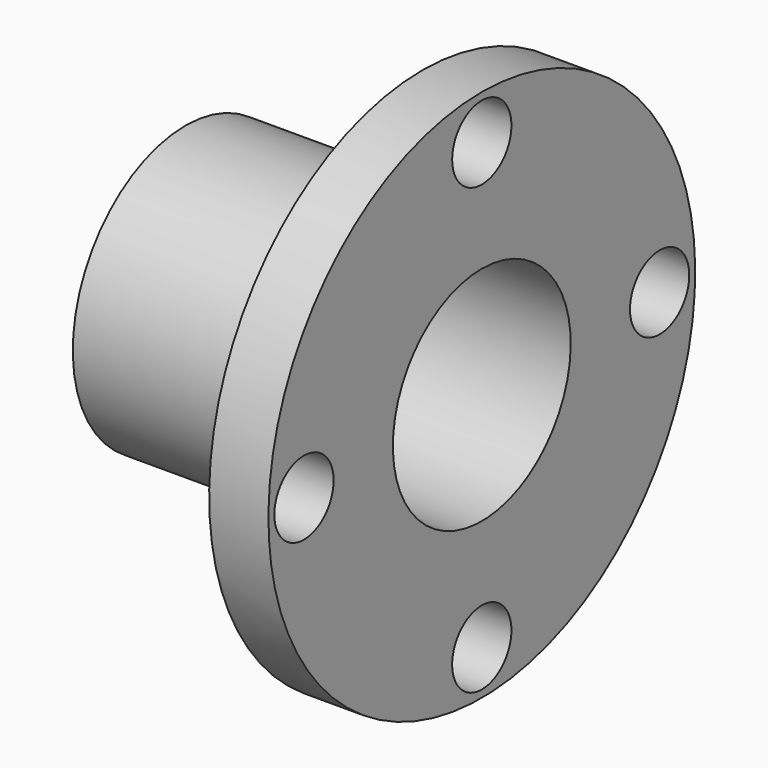
from build123d import *

# Parameters (mm, degrees)
F2_R            = 12.5
F3_DEPTH        = 20.001
F3_COPIES_COUNT = 4


# Not quite as in the source:
# - a pattern or mirror of a feature is missing from the dataset's text; its kind, count and spacing are read off the source's solid


with BuildPart() as f1:
    # F0 (on Front) → F1 (revolve)
    with BuildSketch(Plane.XZ):
        Polygon((-100, 37.5), (0, 37.5), (0, 90), (-20, 90), (-20, 47.5), (-100, 47.5), align=None)
    revolve(axis=Axis((-86.3388044803, 0, 0), (-1, 0, 0)))

    # F2 (on face) → F3 (cut, through all)
    with BuildSketch(Plane(origin=(-20, 0, 0), x_dir=(0, -1, 0), z_dir=(-1, 0, 0))):
        with Locations((0, 75)):
            Circle(F2_R)
    f3 = extrude(amount=-F3_DEPTH, mode=Mode.SUBTRACT)

    # F3_copies: F3 ×4 about axis
    f3_copies_axis = Axis((0, 0, 0), (1, 0, 0))
    for i in range(1, F3_COPIES_COUNT):
        add(f3.rotate(f3_copies_axis, i * 360 / F3_COPIES_COUNT), mode=Mode.SUBTRACT)


solid = f1.part
